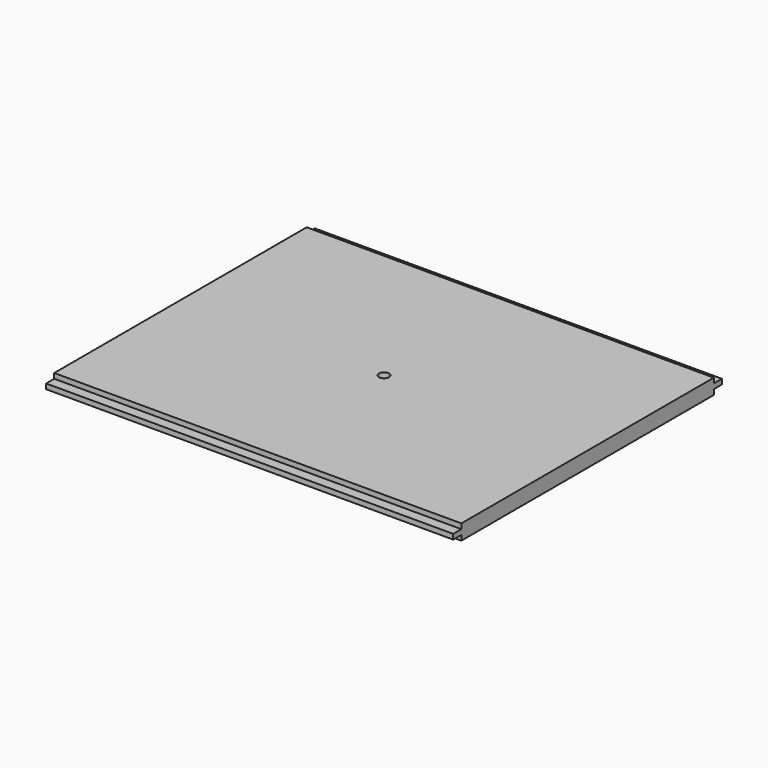
from build123d import *

# Parameters (mm, degrees)
F0_W     = 508
F0_H     = 419.1
F1_DEPTH = 19.05
F2_W     = 508
F2_H     = 6.35
F3_DEPTH = 12.7
F4_R     = 6.35
F5_DEPTH = 19.051


# Not quite as in the source:
# - a pattern or mirror of a feature is missing from the dataset's text; its kind, count and spacing are read off the source's solid


with BuildPart() as f1:
    # F0 (on Top) → F1 (new body)
    with BuildSketch(Plane.XY):
        Rectangle(F0_W, F0_H)
    extrude(amount=F1_DEPTH)

    # F2 (on face) → F3 (cut)
    with BuildSketch(Plane.XZ.offset(209.55)):
        with Locations((0, 3.175)):
            Rectangle(F2_W, F2_H)
        with Locations((0, 15.875)):
            Rectangle(F2_W, F2_H)
    f3 = extrude(amount=-F3_DEPTH, mode=Mode.SUBTRACT)

    # F3_copies: F3 across plane
    add(f3.mirror(Plane.ZX), mode=Mode.SUBTRACT)

    # F4 (on face) → F5 (cut, through all)
    with BuildSketch(Plane.XY.offset(19.05)):
        Circle(F4_R)
    extrude(amount=-F5_DEPTH, mode=Mode.SUBTRACT)


solid = f1.part
